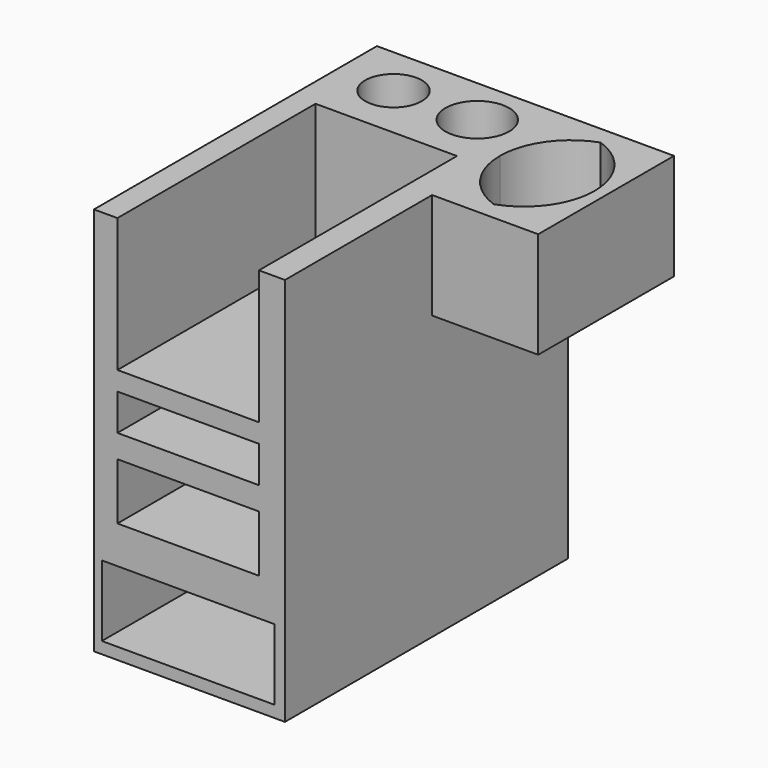
from build123d import *

# Parameters (mm, degrees)
F0_W         = 76.2
F0_H         = 127
F1_DEPTH     = 139.7
F2_R         = 11.43
F3_DEPTH     = 91.44
F4_R         = 10.16
F5_DEPTH     = 133.35
F6_DEPTH     = 12.7
F8_DEPTH     = 5.08
F7_W         = 60.1533111874
F7_H         = 25.4809018224
F7_W_2       = 0.8066888126
F9_DEPTH     = 63.5
F10_DEPTH    = 91.44
F11_R        = 11.43
F12_DEPTH    = 91.44
F13_W        = 60.96
F13_H        = 20.32
F14_DEPTH    = 88.9
F15_DEPTH    = 5.08
F16_DEPTH    = 5.08
F17_W        = 50.8
F17_H        = 12.7
F18_DEPTH    = 86.36
F19_W        = 50.8
F19_H        = 48.0175957203
F20_DEPTH    = 88.9
F21_W        = 6.7573417909
F21_H        = 48.0175957203
F22_DEPTH    = 55.88
F23_W        = 60.96
F23_H        = 38.1
F24_DEPTH    = 38.1
F25_W        = 34.0146065784
F25_H        = 50.826728344
F26_DEPTH    = 50.8
F27_T1_DEPTH = 38.1
F28_DEPTH    = 0.508
F29_DEPTH    = 0.508
F30_DEPTH    = 0.508
F31_DEPTH    = 0.381
F32_DEPTH    = 25.4


# Not quite as in the source:
# - a fillet or chamfer that OpenCascade refuses, or shapes differently, is made with other operations: its cross-section is extruded or revolved along the edge and cut away or added


with BuildPart() as f1:
    # F0 (on Top) → F1 (new body)
    with BuildSketch(Plane.XY):
        with Locations((38.1, 63.5)):
            Rectangle(F0_W, F0_H)
    extrude(amount=F1_DEPTH)

    # F2 (on face) → F3 (cut)
    with BuildSketch(Plane.XY.offset(139.7)):
        with Locations((18.5702368617, 17.6018252969)):
            Circle(F2_R)
    extrude(amount=-F3_DEPTH, mode=Mode.SUBTRACT)

    # F4 (on face) → F5 (cut)
    with BuildSketch(Plane.XY.offset(139.7)):
        with Locations((20.5664373934, 108.7463870645)):
            Circle(F4_R)
    extrude(amount=-F5_DEPTH, mode=Mode.SUBTRACT)

    # F6 (cut): a face of the model
    f6_faces = [f1.faces().sort_by_distance(p)[0] for p in [
        (76.2, 63.5, 69.85),
    ]]
    extrude(f6_faces, amount=-F6_DEPTH, mode=Mode.SUBTRACT)

    # F8 (add): a face of the model
    f8_faces = [f1.faces().sort_by_distance(p)[0] for p in [
        (63.5, 63.5, 69.85),
    ]]
    extrude(f8_faces, amount=F8_DEPTH)

    # F7 (on face) → F9 (cut)
    with BuildSketch(Plane.XZ):
        with Locations((33.4233444063, 16.9386500493)):
            Rectangle(F7_W, F7_H)
        with Locations((63.9033444063, 16.9386500493)):
            Rectangle(F7_W_2, F7_H)
    extrude(amount=-F9_DEPTH, mode=Mode.SUBTRACT)

    # F10 (add): a face of the model
    f10_faces = [f1.faces().sort_by_distance(p)[0] for p in [
        (18.5702368617, 17.6018252969, 48.26),
    ]]
    extrude(f10_faces, amount=F10_DEPTH)

    # F11 (on face) → F12 (cut)
    with BuildSketch(Plane.XY.offset(139.7)):
        with Locations((49.913611263, 109.6450760961)):
            Circle(F11_R)
    extrude(amount=-F12_DEPTH, mode=Mode.SUBTRACT)

    # F13 (on face) → F14 (cut)
    with BuildSketch(Plane.XZ):
        with Locations((33.8266888126, 53.3226364589)):
            Rectangle(F13_W, F13_H)
    extrude(amount=-F14_DEPTH, mode=Mode.SUBTRACT)

    # F15 (add): a face of the model
    f15_faces = [f1.faces().sort_by_distance(p)[0] for p in [
        (3.3466888126, 44.45, 53.3226364589),
    ]]
    extrude(f15_faces, amount=F15_DEPTH)

    # F16 (add): a face of the model
    f16_faces = [f1.faces().sort_by_distance(p)[0] for p in [
        (64.3066888126, 44.45, 53.3226364589),
    ]]
    extrude(f16_faces, amount=F16_DEPTH)

    # F17 (on face) → F18 (cut)
    with BuildSketch(Plane.XZ):
        with Locations((33.8266888126, 78.1391007662)):
            Rectangle(F17_W, F17_H)
    extrude(amount=-F18_DEPTH, mode=Mode.SUBTRACT)

    # F19 (on face) → F20 (cut)
    with BuildSketch(Plane.XZ):
        with Locations((33.8266888126, 115.6912021399)):
            Rectangle(F19_W, F19_H)
    extrude(amount=-F20_DEPTH, mode=Mode.SUBTRACT)

    # F21 (on face) → F22 (join)
    with BuildSketch(Plane.YZ.offset(8.4266888126)):
        with Locations((3.3786708955, 115.6912021399)):
            Rectangle(F21_W, F21_H)
    extrude(amount=F22_DEPTH)

    # F23 (on face) → F24 (join)
    with BuildSketch(Plane.YZ.offset(68.58)):
        with Locations((96.52, 120.65)):
            Rectangle(F23_W, F23_H)
    extrude(amount=F24_DEPTH)

    # F25 (on face) → F26 (cut)
    with BuildSketch(Plane(origin=(0, 0, 101.6), x_dir=(1, 0, 0), z_dir=(0, 0, -1))):
        with Locations((85.5873032892, -96.4670181274)):
            Rectangle(F25_W, F25_H)
    extrude(amount=-F26_DEPTH, mode=Mode.SUBTRACT)

    # F27: fillet of radius 25.4 on 4 edges, made by hand

    # F27_s2 → F27_t1 (join)
    with BuildSketch(Plane.XY.offset(101.6)):
        with BuildLine():
            ThreePointArc((77.1946065784, 71.0536539555), (95.1551188205, 78.4931417133), (102.5946065784, 96.4536539555))
            Line((102.5946065784, 96.4536539555), (102.5946065784, 71.0536539555))
            Line((102.5946065784, 71.0536539555), (77.1946065784, 71.0536539555))
        make_face()
        with BuildLine():
            ThreePointArc((102.5946065784, 96.4803822994), (95.1551188205, 114.4408945416), (77.1946065784, 121.8803822994))
            Line((77.1946065784, 121.8803822994), (102.5946065784, 121.8803822994))
            Line((102.5946065784, 121.8803822994), (102.5946065784, 96.4803822994))
        make_face()
        with BuildLine():
            ThreePointArc((68.58, 96.4536539555), (76.0194877579, 78.4931417133), (93.98, 71.0536539555))
            Line((93.98, 71.0536539555), (68.58, 71.0536539555))
            Line((68.58, 71.0536539555), (68.58, 96.4536539555))
        make_face()
        with BuildLine():
            ThreePointArc((68.58, 96.4803822994), (76.0194877579, 114.4408945416), (93.98, 121.8803822994))
            Line((93.98, 121.8803822994), (68.58, 121.8803822994))
            Line((68.58, 121.8803822994), (68.58, 96.4803822994))
        make_face()
    extrude(amount=F27_T1_DEPTH)

    # F28 (cut): a face of the model
    f28_faces = [f1.faces().sort_by_distance(p)[0] for p in [
        (33.8266888126, 63.5, 16.9386500493),
    ]]
    extrude(f28_faces, amount=-F28_DEPTH, mode=Mode.SUBTRACT)

    # F29 (cut): a face of the model
    f29_faces = [f1.faces().sort_by_distance(p)[0] for p in [
        (3.3466888126, 32.004, 16.9386500493),
    ]]
    extrude(f29_faces, amount=-F29_DEPTH, mode=Mode.SUBTRACT)

    # F30 (cut): a face of the model
    f30_faces = [f1.faces().sort_by_distance(p)[0] for p in [
        (64.3066888126, 32.004, 16.9386500493),
    ]]
    extrude(f30_faces, amount=-F30_DEPTH, mode=Mode.SUBTRACT)

    # F31 (cut): a face of the model
    f31_faces = [f1.faces().sort_by_distance(p)[0] for p in [
        (33.8266888126, 43.18, 84.4891007662),
    ]]
    extrude(f31_faces, amount=-F31_DEPTH, mode=Mode.SUBTRACT)

    # F32 (cut): a face of the model
    f32_faces = [f1.faces().sort_by_distance(p)[0] for p in [
        (33.8266888126, 6.7573417909, 115.6912021399),
    ]]
    extrude(f32_faces, amount=-F32_DEPTH, mode=Mode.SUBTRACT)


solid = f1.part
